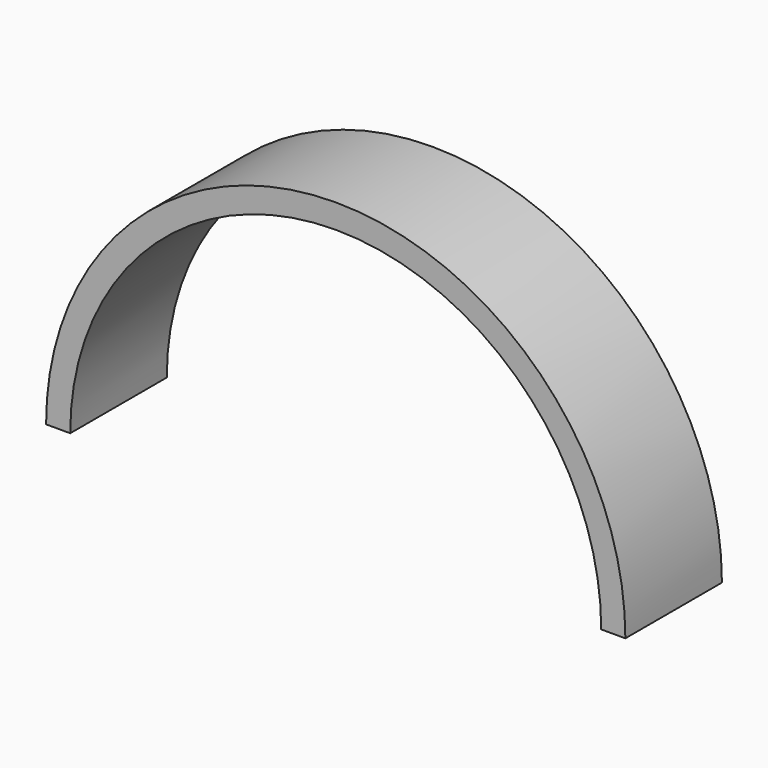
from build123d import *

# Parameters (mm, degrees)
F1_DEPTH = 25


# Not quite as in the source:
# - a feature names something its author has since deleted; it is built from what else it names


with BuildPart() as f1:
    # F0 (on Front) → F1 (new body)
    with BuildSketch(Plane.XZ):
        with BuildLine():
            Line((55, 0), (60, 0))
            ThreePointArc((60, 0), (0, 60), (-60, 0))
            Line((-60, 0), (-55, 0))
            ThreePointArc((-55, 0), (0, 55), (55, 0))
        make_face()
    extrude(amount=F1_DEPTH)


solid = f1.part
